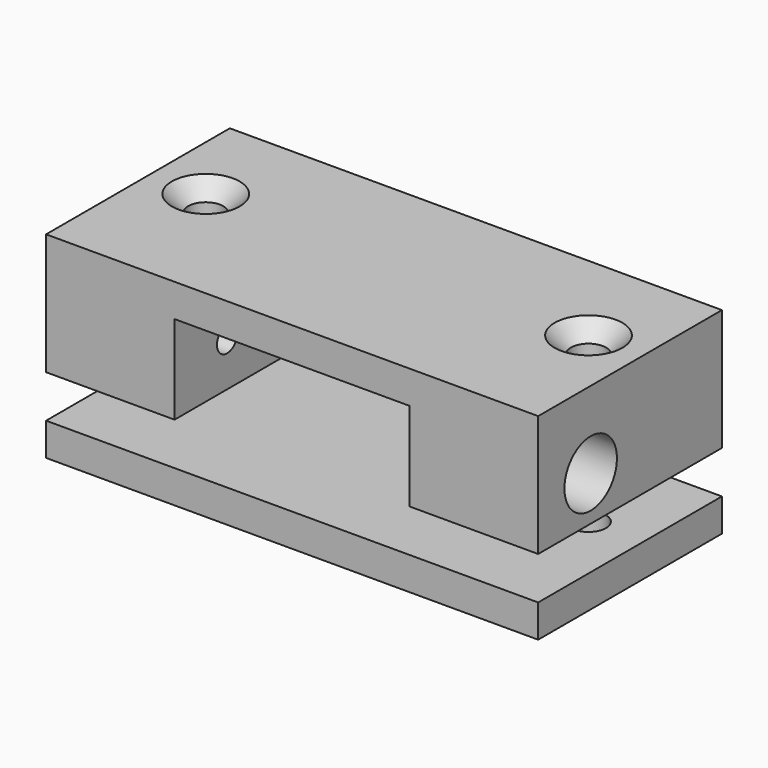
from build123d import *

# Parameters (mm, degrees)
F0_R     = 1.6
F1_DEPTH = 3
F3_DEPTH = 8.1
F4_SIZE  = 1.5
F5_R     = 1.15
F6_DEPTH = 45.001
F5_R_2   = 3
F7_DEPTH = 4


# Not quite as in the source:
# - a pattern or mirror of a feature is missing from the dataset's text; its kind, count and spacing are read off the source's solid


with BuildPart() as f1:
    # F0 (on Top) → F1 (new body)
    with BuildSketch(Plane.XY):
        Polygon((-10.75, -12), (10.75, -12), (10.75, 0), (12.5, 0), (12.5, 1.5), (11.75, 1.5), (11.75, 9), (-11.75, 9), (-11.75, 1.5), (-12.5, 1.5), (-12.5, 0), (-10.75, 0), align=None)
        Polygon((10.75, 0), (10.75, -12), (22.5, -12), (22.5, 9), (11.75, 9), (11.75, 1.5), (12.5, 1.5), (12.5, 0), align=None)
        with Locations((17.5, 0)):
            Circle(F0_R, mode=Mode.SUBTRACT)
        Polygon((-22.5, -12), (-10.75, -12), (-10.75, 0), (-12.5, 0), (-12.5, 1.5), (-11.75, 1.5), (-11.75, 9), (-22.5, 9), align=None)
        with Locations((-17.5, 0)):
            Circle(F0_R, mode=Mode.SUBTRACT)
    extrude(amount=F1_DEPTH)


with BuildPart() as f2_1:
    # F2: copy of F1
    add(f1.part.moved(Location((0, 0, -15))))


with BuildPart() as f1_1:
    add(f1.part)

    # F0 (on Top) → F3 (join)
    with BuildSketch(Plane.XY):
        Polygon((-22.5, -12), (-10.75, -12), (-10.75, 0), (-12.5, 0), (-12.5, 1.5), (-11.75, 1.5), (-11.75, 9), (-22.5, 9), align=None)
        with Locations((-17.5, 0)):
            Circle(F0_R, mode=Mode.SUBTRACT)
        Polygon((10.75, 0), (10.75, -12), (22.5, -12), (22.5, 9), (11.75, 9), (11.75, 1.5), (12.5, 1.5), (12.5, 0), align=None)
        with Locations((17.5, 0)):
            Circle(F0_R, mode=Mode.SUBTRACT)
    extrude(amount=-F3_DEPTH)

    # F4
    f4_edges = [f1_1.edges().sort_by_distance(p)[0] for p in [
        (-19.1, 0, 3),
        (15.9, 0, 3),
    ]]
    chamfer(f4_edges, length=F4_SIZE)

    # F5 (on face) → F6 (cut, through all)
    with BuildSketch(Plane(origin=(-22.5, 0, 0), x_dir=(0, -1, 0), z_dir=(-1, 0, 0))):
        with Locations((6, -4.05)):
            Circle(F5_R)
    extrude(amount=-F6_DEPTH, mode=Mode.SUBTRACT)

    # F5 (on face) → F7 (cut)
    with BuildSketch(Plane(origin=(-22.5, 0, 0), x_dir=(0, -1, 0), z_dir=(-1, 0, 0))):
        with Locations((6, -4.05)):
            Circle(F5_R_2)
        with Locations((6, -4.05)):
            Circle(F5_R, mode=Mode.SUBTRACT)
    f7 = extrude(amount=-F7_DEPTH, mode=Mode.SUBTRACT)

    # F7_copies: F7 across plane
    add(f7.mirror(Plane(origin=(0, 0, 0), x_dir=(0, 0, 1), z_dir=(1, 0, 0))), mode=Mode.SUBTRACT)


solid = Compound([f2_1.part, f1_1.part])
